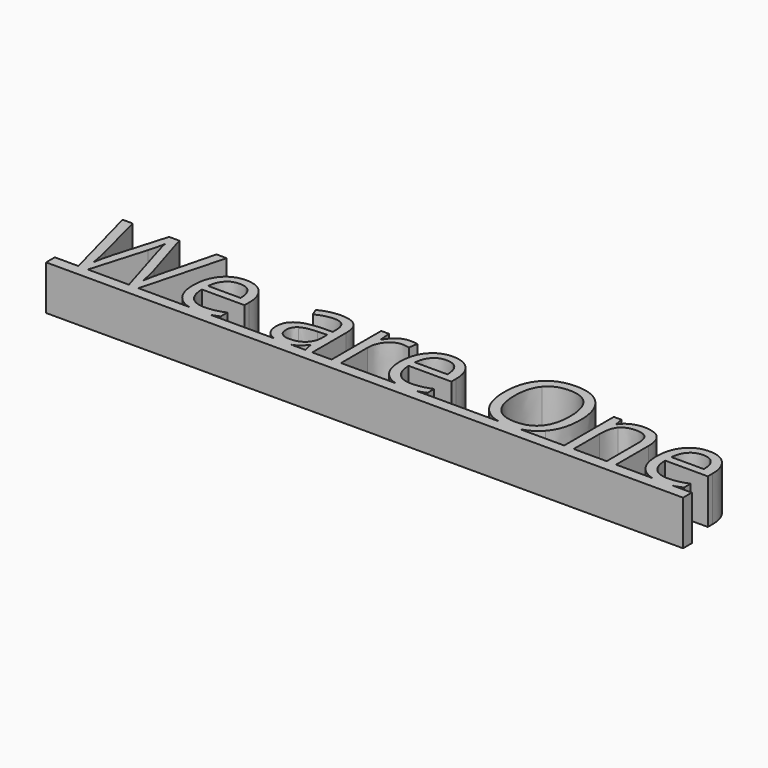
from build123d import *

# Parameters (mm, degrees)
F1_DEPTH = 7


with BuildPart() as f1:
    # F0 (on Top) → F1 (new body)
    with BuildSketch(Plane.XY):
        with BuildLine():
            Line((39.0246675003, -11.7085370013), (39.3173809253, -13.0953734228))
            Line((39.3173809253, -13.0953734228), (40.4115039218, -13.0953734228))
            Line((40.4115039218, -13.0953734228), (40.4115039218, -6.4510628623))
            add(Edge.make_bspline(
                [(39.5717289985, -3.9743662612), (40.4115039218, -4.7459361146), (40.4115039218, -6.4510628623)],
                knots=[0, 0, 0, 1, 1, 1], degree=2))
            add(Edge.make_bspline(
                [(36.9927247925, -3.2027964079), (38.7319540753, -3.2027964079), (39.5717289985, -3.9743662612)],
                knots=[0, 0, 0, 1, 1, 1], degree=2))
            add(Edge.make_bspline(
                [(35.2719677163, -3.4244628851), (36.128793907, -3.2027964079), (36.9927247925, -3.2027964079)],
                knots=[0, 0, 0, 1, 1, 1], degree=2))
            add(Edge.make_bspline(
                [(33.6961464136, -4.0354666364), (34.4151415255, -3.6461293623), (35.2719677163, -3.4244628851)],
                knots=[0, 0, 0, 1, 1, 1], degree=2))
            Line((33.6961464136, -4.0354666364), (34.1508468796, -5.1636921678))
            add(Edge.make_bspline(
                [(36.9017846993, -4.4191201546), (35.6854609526, -4.4191201546), (34.1508468796, -5.1636921678)],
                knots=[0, 0, 0, 1, 1, 1], degree=2))
            add(Edge.make_bspline(
                [(38.479026941, -4.9647607139), (37.9873820621, -4.4191201546), (36.9017846993, -4.4191201546)],
                knots=[0, 0, 0, 1, 1, 1], degree=2))
            add(Edge.make_bspline(
                [(38.9706718199, -6.6556780721), (38.9706718199, -5.5104012732), (38.479026941, -4.9647607139)],
                knots=[0, 0, 0, 1, 1, 1], degree=2))
            Line((38.9706718199, -6.6556780721), (38.9706718199, -7.2609980675))
            Line((38.9706718199, -7.2609980675), (37.3195407525, -7.3149937479))
            add(Edge.make_bspline(
                [(32.604865295, -10.4041150392), (32.604865295, -7.4570876435), (37.3195407525, -7.3149937479)],
                knots=[0, 0, 0, 1, 1, 1], degree=2))
            add(Edge.make_bspline(
                [(33.4261680118, -12.5269978402), (32.604865295, -11.7795839491), (32.604865295, -10.4041150392)],
                knots=[0, 0, 0, 1, 1, 1], degree=2))
            add(Edge.make_bspline(
                [(34.4278100444, -13.0953734228), (33.8454988608, -12.9086034224), (33.4261680118, -12.5269978402)],
                knots=[0.4894320446, 0.4894320446, 0.4894320446, 1, 1, 1], degree=2))
            Line((34.4278100444, -13.0953734228), (37.1051414676, -13.0953734228))
            add(Edge.make_bspline(
                [(37.5028418779, -12.9490167102), (37.3160728416, -13.0330444299), (37.1051414676, -13.0953734228)],
                knots=[0, 0, 0, 0.2582329607, 0.2582329607, 0.2582329607], degree=2))
            add(Edge.make_bspline(
                [(38.9536205525, -11.7085370013), (38.2260998068, -12.6236216892), (37.5028418779, -12.9490167102)],
                knots=[0, 0, 0, 1, 1, 1], degree=2))
            Line((38.9536205525, -11.7085370013), (39.0246675003, -11.7085370013))
        make_face()
        with BuildLine():
            add(Edge.make_bspline(
                [(35.9867000114, -12.0552461066), (37.3650107991, -12.0552461066), (38.1507900421, -11.3007275207)],
                knots=[0, 0, 0, 1, 1, 1], degree=2))
            add(Edge.make_bspline(
                [(34.6339661248, -11.6389109924), (35.11708537, -12.0552461066), (35.9867000114, -12.0552461066)],
                knots=[0, 0, 0, 1, 1, 1], degree=2))
            add(Edge.make_bspline(
                [(34.1508468796, -10.4211663067), (34.1508468796, -11.2225758781), (34.6339661248, -11.6389109924)],
                knots=[0, 0, 0, 1, 1, 1], degree=2))
            add(Edge.make_bspline(
                [(34.9266795498, -8.9163919518), (34.1508468796, -9.400932136), (34.1508468796, -10.4211663067)],
                knots=[0, 0, 0, 1, 1, 1], degree=2))
            add(Edge.make_bspline(
                [(37.4616346482, -8.3693304536), (35.7025122201, -8.4318517676), (34.9266795498, -8.9163919518)],
                knots=[0, 0, 0, 1, 1, 1], degree=2))
            Line((37.4616346482, -8.3693304536), (38.936569285, -8.3096510174))
            Line((38.936569285, -8.3096510174), (38.936569285, -9.1877912925))
            add(Edge.make_bspline(
                [(38.1507900421, -11.3007275207), (38.936569285, -10.5462089349), (38.936569285, -9.1877912925)],
                knots=[0, 0, 0, 1, 1, 1], degree=2))
        make_face(mode=Mode.SUBTRACT)
        with BuildLine():
            Line((40.4115039218, -13.0953734228), (39.3173809253, -13.0953734228))
            Line((39.3173809253, -13.0953734228), (37.1051414676, -13.0953734228))
            add(Edge.make_bspline(
                [(37.1051414676, -13.0953734228), (36.499246928, -13.2744117313), (35.6939865863, -13.2744117313)],
                knots=[0.2582329607, 0.2582329607, 0.2582329607, 1, 1, 1], degree=2))
            add(Edge.make_bspline(
                [(35.6939865863, -13.2744117313), (34.9860153726, -13.2744117313), (34.4278100444, -13.0953734228)],
                knots=[0, 0, 0, 0.4894320446, 0.4894320446, 0.4894320446], degree=2))
            Line((34.4278100444, -13.0953734228), (24.3351313223, -13.0953734228))
            add(Edge.make_bspline(
                [(24.3351313223, -13.0953734228), (24.2650180095, -13.1119319906), (24.1957485506, -13.1266340798)],
                knots=[0.9005120931, 0.9005120931, 0.9005120931, 1, 1, 1], degree=2))
            add(Edge.make_bspline(
                [(24.1957485506, -13.1266340798), (23.499488462, -13.2744117313), (22.5133568262, -13.2744117313)],
                knots=[0, 0, 0, 1, 1, 1], degree=2))
            add(Edge.make_bspline(
                [(22.5133568262, -13.2744117313), (21.7176978405, -13.2744117313), (21.0455868884, -13.0953734228)],
                knots=[0, 0, 0, 0.3688754729, 0.3688754729, 0.3688754729], degree=2))
            Line((21.0455868884, -13.0953734228), (15.2645353461, -13.0953734228))
            Line((15.2645353461, -13.0953734228), (13.1181084461, -13.0953734228))
            Line((13.1181084461, -13.0953734228), (11.6261225418, -13.0953734228))
            Line((11.6261225418, -13.0953734228), (5.1864271911, -13.0953734228))
            Line((5.1864271911, -13.0953734228), (3.6944412868, -13.0953734228))
            Line((3.6944412868, -13.0953734228), (0, -13.0953734228))
            Line((0, -13.0953734228), (0, -14.8112857714))
            Line((0, -14.8112857714), (99.9942272902, -14.8112857714))
            Line((99.9942272902, -14.8112857714), (99.9942272902, -13.0953734228))
            Line((99.9942272902, -13.0953734228), (97.0644708699, -13.0953734228))
            add(Edge.make_bspline(
                [(97.0644708699, -13.0953734228), (96.9943575571, -13.1119319906), (96.9250880982, -13.1266340798)],
                knots=[0.9005120931, 0.9005120931, 0.9005120931, 1, 1, 1], degree=2))
            add(Edge.make_bspline(
                [(96.9250880982, -13.1266340798), (96.2288280095, -13.2744117313), (95.2426963738, -13.2744117313)],
                knots=[0, 0, 0, 1, 1, 1], degree=2))
            add(Edge.make_bspline(
                [(95.2426963738, -13.2744117313), (94.447037388, -13.2744117313), (93.774926436, -13.0953734228)],
                knots=[0, 0, 0, 0.3688754729, 0.3688754729, 0.3688754729], degree=2))
            Line((93.774926436, -13.0953734228), (88.1038990565, -13.0953734228))
            Line((88.1038990565, -13.0953734228), (86.6289644197, -13.0953734228))
            Line((86.6289644197, -13.0953734228), (86.2403680865, -13.0953734228))
            Line((86.2403680865, -13.0953734228), (81.4425372286, -13.0953734228))
            Line((81.4425372286, -13.0953734228), (79.9676025918, -13.0953734228))
            Line((79.9676025918, -13.0953734228), (72.9898686268, -13.0953734228))
            add(Edge.make_bspline(
                [(72.9898686268, -13.0953734228), (72.224875064, -13.2744117313), (71.3368193702, -13.2744117313)],
                knots=[0.6833950988, 0.6833950988, 0.6833950988, 1, 1, 1], degree=2))
            add(Edge.make_bspline(
                [(71.3368193702, -13.2744117313), (70.4209187003, -13.2744117313), (69.6385356677, -13.0953734228)],
                knots=[0, 0, 0, 0.319412416, 0.319412416, 0.319412416], degree=2))
            Line((69.6385356677, -13.0953734228), (56.8064283554, -13.0953734228))
            add(Edge.make_bspline(
                [(56.8064283554, -13.0953734228), (56.7363150426, -13.1119319906), (56.6670455837, -13.1266340798)],
                knots=[0.9005120931, 0.9005120931, 0.9005120931, 1, 1, 1], degree=2))
            add(Edge.make_bspline(
                [(56.6670455837, -13.1266340798), (55.9707854951, -13.2744117313), (54.9846538593, -13.2744117313)],
                knots=[0, 0, 0, 1, 1, 1], degree=2))
            add(Edge.make_bspline(
                [(54.9846538593, -13.2744117313), (54.1889948736, -13.2744117313), (53.5168839215, -13.0953734228)],
                knots=[0, 0, 0, 0.3688754729, 0.3688754729, 0.3688754729], degree=2))
            Line((53.5168839215, -13.0953734228), (44.9215641696, -13.0953734228))
            Line((44.9215641696, -13.0953734228), (43.4466295328, -13.0953734228))
            Line((43.4466295328, -13.0953734228), (40.4115039218, -13.0953734228))
        make_face()
        with BuildLine():
            add(Edge.make_bspline(
                [(37.1051414676, -13.0953734228), (36.499246928, -13.2744117313), (35.6939865863, -13.2744117313)],
                knots=[0.2582329607, 0.2582329607, 0.2582329607, 1, 1, 1], degree=2))
            Line((37.1051414676, -13.0953734228), (34.4278100444, -13.0953734228))
            add(Edge.make_bspline(
                [(35.6939865863, -13.2744117313), (34.9860153726, -13.2744117313), (34.4278100444, -13.0953734228)],
                knots=[0, 0, 0, 0.4894320446, 0.4894320446, 0.4894320446], degree=2))
        make_face()
        with BuildLine():
            Line((43.4466295328, -3.361941571), (43.4466295328, -13.0953734228))
            Line((43.4466295328, -13.0953734228), (44.9215641696, -13.0953734228))
            Line((44.9215641696, -13.0953734228), (44.9215641696, -7.8720018188))
            add(Edge.make_bspline(
                [(45.7599181539, -5.483403433), (44.9215641696, -6.4425372286), (44.9215641696, -7.8720018188)],
                knots=[0, 0, 0, 1, 1, 1], degree=2))
            add(Edge.make_bspline(
                [(47.78049335, -4.5242696374), (46.5982721382, -4.5242696374), (45.7599181539, -5.483403433)],
                knots=[0, 0, 0, 1, 1, 1], degree=2))
            add(Edge.make_bspline(
                [(48.8461975674, -4.6578378993), (48.2437194498, -4.5242696374), (47.78049335, -4.5242696374)],
                knots=[0, 0, 0, 1, 1, 1], degree=2))
            Line((48.8461975674, -4.6578378993), (49.0508127771, -3.2908946232))
            add(Edge.make_bspline(
                [(47.8884847107, -3.1829032625), (48.5364328748, -3.1829032625), (49.0508127771, -3.2908946232)],
                knots=[0, 0, 0, 1, 1, 1], degree=2))
            add(Edge.make_bspline(
                [(46.2089348642, -3.6987041037), (46.9734000227, -3.1829032625), (47.8884847107, -3.1829032625)],
                knots=[0, 0, 0, 1, 1, 1], degree=2))
            add(Edge.make_bspline(
                [(44.9045129021, -5.1636921678), (45.4444697056, -4.2145049449), (46.2089348642, -3.6987041037)],
                knots=[0, 0, 0, 1, 1, 1], degree=2))
            Line((44.9045129021, -5.1636921678), (44.8334659543, -5.1636921678))
            Line((44.8334659543, -5.1636921678), (44.6629532795, -3.361941571))
            Line((44.6629532795, -3.361941571), (43.4466295328, -3.361941571))
        make_face()
        with BuildLine():
            add(Edge.make_bspline(
                [(24.3351313223, -13.0953734228), (24.2650180095, -13.1119319906), (24.1957485506, -13.1266340798)],
                knots=[0.9005120931, 0.9005120931, 0.9005120931, 1, 1, 1], degree=2))
            Line((24.3351313223, -13.0953734228), (21.0455868884, -13.0953734228))
            add(Edge.make_bspline(
                [(22.5133568262, -13.2744117313), (21.7176978405, -13.2744117313), (21.0455868884, -13.0953734228)],
                knots=[0, 0, 0, 0.3688754729, 0.3688754729, 0.3688754729], degree=2))
            add(Edge.make_bspline(
                [(24.1957485506, -13.1266340798), (23.499488462, -13.2744117313), (22.5133568262, -13.2744117313)],
                knots=[0, 0, 0, 1, 1, 1], degree=2))
        make_face()
        with BuildLine():
            Line((21.0455868884, -13.0953734228), (24.3351313223, -13.0953734228))
            add(Edge.make_bspline(
                [(25.6735250654, -12.6435148346), (24.9697600728, -12.9454939951), (24.3351313223, -13.0953734228)],
                knots=[0, 0, 0, 0.9005120931, 0.9005120931, 0.9005120931], degree=2))
            Line((25.6735250654, -12.6435148346), (25.6735250654, -11.3277253609))
            add(Edge.make_bspline(
                [(22.5673525065, -11.9841991588), (24.1389109924, -11.9841991588), (25.6735250654, -11.3277253609)],
                knots=[0, 0, 0, 1, 1, 1], degree=2))
            add(Edge.make_bspline(
                [(20.2540638854, -11.096112311), (21.0753666023, -11.9841991588), (22.5673525065, -11.9841991588)],
                knots=[0, 0, 0, 1, 1, 1], degree=2))
            add(Edge.make_bspline(
                [(19.387291122, -8.4943730817), (19.4327611686, -10.2080254632), (20.2540638854, -11.096112311)],
                knots=[0, 0, 0, 1, 1, 1], degree=2))
            Line((19.387291122, -8.4943730817), (26.0912811186, -8.4943730817))
            Line((26.0912811186, -8.4943730817), (26.0912811186, -7.5622371263))
            add(Edge.make_bspline(
                [(25.0255769012, -4.3864385586), (26.0912811186, -5.5899738547), (26.0912811186, -7.5622371263)],
                knots=[0, 0, 0, 1, 1, 1], degree=2))
            add(Edge.make_bspline(
                [(22.1325451859, -3.1829032625), (23.9598726839, -3.1829032625), (25.0255769012, -4.3864385586)],
                knots=[0, 0, 0, 1, 1, 1], degree=2))
            add(Edge.make_bspline(
                [(19.0178469933, -4.568318745), (20.1773331818, -3.1829032625), (22.1325451859, -3.1829032625)],
                knots=[0, 0, 0, 1, 1, 1], degree=2))
            add(Edge.make_bspline(
                [(17.8583608048, -8.3096510174), (17.8583608048, -5.9537342276), (19.0178469933, -4.568318745)],
                knots=[0, 0, 0, 1, 1, 1], degree=2))
            add(Edge.make_bspline(
                [(19.1073661476, -11.9586222576), (17.8583608048, -10.6428327839), (17.8583608048, -8.3096510174)],
                knots=[0, 0, 0, 1, 1, 1], degree=2))
            add(Edge.make_bspline(
                [(21.0455868884, -13.0953734228), (19.8956440539, -12.789049267), (19.1073661476, -11.9586222576)],
                knots=[0.3688754729, 0.3688754729, 0.3688754729, 1, 1, 1], degree=2))
        make_face()
        with BuildLine():
            add(Edge.make_bspline(
                [(22.1126520405, -4.4191201546), (20.9417983403, -4.4191201546), (20.2441173127, -5.1821643742)],
                knots=[0, 0, 0, 1, 1, 1], degree=2))
            add(Edge.make_bspline(
                [(23.890246675, -5.1608502899), (23.269296351, -4.4191201546), (22.1126520405, -4.4191201546)],
                knots=[0, 0, 0, 1, 1, 1], degree=2))
            add(Edge.make_bspline(
                [(24.511196999, -7.2951006025), (24.511196999, -5.9025804251), (23.890246675, -5.1608502899)],
                knots=[0, 0, 0, 1, 1, 1], degree=2))
            Line((24.511196999, -7.2951006025), (19.4213936569, -7.2951006025))
            add(Edge.make_bspline(
                [(20.2441173127, -5.1821643742), (19.5464362851, -5.9452085938), (19.4213936569, -7.2951006025)],
                knots=[0, 0, 0, 1, 1, 1], degree=2))
        make_face(mode=Mode.SUBTRACT)
        with BuildLine():
            add(Edge.make_bspline(
                [(53.5168839215, -13.0953734228), (52.366941087, -12.789049267), (51.5786631806, -11.9586222576)],
                knots=[0.3688754729, 0.3688754729, 0.3688754729, 1, 1, 1], degree=2))
            Line((53.5168839215, -13.0953734228), (56.8064283554, -13.0953734228))
            add(Edge.make_bspline(
                [(58.1448220984, -12.6435148346), (57.4410571058, -12.9454939951), (56.8064283554, -13.0953734228)],
                knots=[0, 0, 0, 0.9005120931, 0.9005120931, 0.9005120931], degree=2))
            Line((58.1448220984, -12.6435148346), (58.1448220984, -11.3277253609))
            add(Edge.make_bspline(
                [(55.0386495396, -11.9841991588), (56.6102080255, -11.9841991588), (58.1448220984, -11.3277253609)],
                knots=[0, 0, 0, 1, 1, 1], degree=2))
            add(Edge.make_bspline(
                [(52.7253609185, -11.096112311), (53.5466636353, -11.9841991588), (55.0386495396, -11.9841991588)],
                knots=[0, 0, 0, 1, 1, 1], degree=2))
            add(Edge.make_bspline(
                [(51.8585881551, -8.4943730817), (51.9040582017, -10.2080254632), (52.7253609185, -11.096112311)],
                knots=[0, 0, 0, 1, 1, 1], degree=2))
            Line((51.8585881551, -8.4943730817), (58.5625781516, -8.4943730817))
            Line((58.5625781516, -8.4943730817), (58.5625781516, -7.5622371263))
            add(Edge.make_bspline(
                [(57.4968739343, -4.3864385586), (58.5625781516, -5.5899738547), (58.5625781516, -7.5622371263)],
                knots=[0, 0, 0, 1, 1, 1], degree=2))
            add(Edge.make_bspline(
                [(54.6038422189, -3.1829032625), (56.4311697169, -3.1829032625), (57.4968739343, -4.3864385586)],
                knots=[0, 0, 0, 1, 1, 1], degree=2))
            add(Edge.make_bspline(
                [(51.4891440264, -4.568318745), (52.6486302148, -3.1829032625), (54.6038422189, -3.1829032625)],
                knots=[0, 0, 0, 1, 1, 1], degree=2))
            add(Edge.make_bspline(
                [(50.3296578379, -8.3096510174), (50.3296578379, -5.9537342276), (51.4891440264, -4.568318745)],
                knots=[0, 0, 0, 1, 1, 1], degree=2))
            add(Edge.make_bspline(
                [(51.5786631806, -11.9586222576), (50.3296578379, -10.6428327839), (50.3296578379, -8.3096510174)],
                knots=[0, 0, 0, 1, 1, 1], degree=2))
        make_face()
        with BuildLine():
            add(Edge.make_bspline(
                [(54.5839490735, -4.4191201546), (53.4130953734, -4.4191201546), (52.7154143458, -5.1821643742)],
                knots=[0, 0, 0, 1, 1, 1], degree=2))
            add(Edge.make_bspline(
                [(56.3615437081, -5.1608502899), (55.7405933841, -4.4191201546), (54.5839490735, -4.4191201546)],
                knots=[0, 0, 0, 1, 1, 1], degree=2))
            add(Edge.make_bspline(
                [(56.9824940321, -7.2951006025), (56.9824940321, -5.9025804251), (56.3615437081, -5.1608502899)],
                knots=[0, 0, 0, 1, 1, 1], degree=2))
            Line((56.9824940321, -7.2951006025), (51.89269069, -7.2951006025))
            add(Edge.make_bspline(
                [(52.7154143458, -5.1821643742), (52.0177333182, -5.9452085938), (51.89269069, -7.2951006025)],
                knots=[0, 0, 0, 1, 1, 1], degree=2))
        make_face(mode=Mode.SUBTRACT)
        with BuildLine():
            Line((56.8064283554, -13.0953734228), (53.5168839215, -13.0953734228))
            add(Edge.make_bspline(
                [(54.9846538593, -13.2744117313), (54.1889948736, -13.2744117313), (53.5168839215, -13.0953734228)],
                knots=[0, 0, 0, 0.3688754729, 0.3688754729, 0.3688754729], degree=2))
            add(Edge.make_bspline(
                [(56.6670455837, -13.1266340798), (55.9707854951, -13.2744117313), (54.9846538593, -13.2744117313)],
                knots=[0, 0, 0, 1, 1, 1], degree=2))
            add(Edge.make_bspline(
                [(56.8064283554, -13.0953734228), (56.7363150426, -13.1119319906), (56.6670455837, -13.1266340798)],
                knots=[0.9005120931, 0.9005120931, 0.9005120931, 1, 1, 1], degree=2))
        make_face()
        with BuildLine():
            add(Edge.make_bspline(
                [(69.6385356677, -13.0953734228), (67.9714740531, -12.7138877831), (66.9105945209, -11.51955212)],
                knots=[0.319412416, 0.319412416, 0.319412416, 1, 1, 1], degree=2))
            Line((69.6385356677, -13.0953734228), (72.9898686268, -13.0953734228))
            add(Edge.make_bspline(
                [(75.718995112, -11.488291463), (74.6411154944, -12.7089173001), (72.9898686268, -13.0953734228)],
                knots=[0, 0, 0, 0.6833950988, 0.6833950988, 0.6833950988], degree=2))
            add(Edge.make_bspline(
                [(77.2962373536, -6.5846311242), (77.2962373536, -9.7021711947), (75.718995112, -11.488291463)],
                knots=[0, 0, 0, 1, 1, 1], degree=2))
            add(Edge.make_bspline(
                [(75.7246788678, -1.6823917245), (77.2962373536, -3.45856542), (77.2962373536, -6.5846311242)],
                knots=[0, 0, 0, 1, 1, 1], degree=2))
            add(Edge.make_bspline(
                [(71.3538706377, 0.0937819711), (74.1531203819, 0.0937819711), (75.7246788678, -1.6823917245)],
                knots=[0, 0, 0, 1, 1, 1], degree=2))
            add(Edge.make_bspline(
                [(66.9148573377, -1.6511310674), (68.4778901898, 0.0937819711), (71.3538706377, 0.0937819711)],
                knots=[0, 0, 0, 1, 1, 1], degree=2))
            add(Edge.make_bspline(
                [(65.3518244856, -6.5675798568), (65.3518244856, -3.3960441059), (66.9148573377, -1.6511310674)],
                knots=[0, 0, 0, 1, 1, 1], degree=2))
            add(Edge.make_bspline(
                [(66.9105945209, -11.51955212), (65.3518244856, -9.7646925088), (65.3518244856, -6.5675798568)],
                knots=[0, 0, 0, 1, 1, 1], degree=2))
        make_face()
        with BuildLine():
            add(Edge.make_bspline(
                [(66.9489598727, -6.5846311242), (66.9489598727, -9.2218938274), (68.0729225872, -10.5859952256)],
                knots=[0, 0, 0, 1, 1, 1], degree=2))
            add(Edge.make_bspline(
                [(68.0729225872, -2.6202114357), (66.9489598727, -3.9843128339), (66.9489598727, -6.5846311242)],
                knots=[0, 0, 0, 1, 1, 1], degree=2))
            add(Edge.make_bspline(
                [(71.3538706377, -1.2561100375), (69.1968853018, -1.2561100375), (68.0729225872, -2.6202114357)],
                knots=[0, 0, 0, 1, 1, 1], degree=2))
            add(Edge.make_bspline(
                [(74.5992952143, -2.610264863), (73.5023303399, -1.2561100375), (71.3538706377, -1.2561100375)],
                knots=[0, 0, 0, 1, 1, 1], degree=2))
            add(Edge.make_bspline(
                [(75.6962600887, -6.5846311242), (75.6962600887, -3.9644196885), (74.5992952143, -2.610264863)],
                knots=[0, 0, 0, 1, 1, 1], degree=2))
            add(Edge.make_bspline(
                [(74.5950323974, -10.5916789815), (75.6962600887, -9.2332613391), (75.6962600887, -6.5846311242)],
                knots=[0, 0, 0, 1, 1, 1], degree=2))
            add(Edge.make_bspline(
                [(71.3368193702, -11.9500966238), (73.4938047061, -11.9500966238), (74.5950323974, -10.5916789815)],
                knots=[0, 0, 0, 1, 1, 1], degree=2))
            add(Edge.make_bspline(
                [(68.0729225872, -10.5859952256), (69.1968853018, -11.9500966238), (71.3368193702, -11.9500966238)],
                knots=[0, 0, 0, 1, 1, 1], degree=2))
        make_face(mode=Mode.SUBTRACT)
        with BuildLine():
            Line((72.9898686268, -13.0953734228), (69.6385356677, -13.0953734228))
            add(Edge.make_bspline(
                [(71.3368193702, -13.2744117313), (70.4209187003, -13.2744117313), (69.6385356677, -13.0953734228)],
                knots=[0, 0, 0, 0.319412416, 0.319412416, 0.319412416], degree=2))
            add(Edge.make_bspline(
                [(72.9898686268, -13.0953734228), (72.224875064, -13.2744117313), (71.3368193702, -13.2744117313)],
                knots=[0.6833950988, 0.6833950988, 0.6833950988, 1, 1, 1], degree=2))
        make_face()
        with BuildLine():
            Line((11.6261225418, -13.0953734228), (13.1181084461, -13.0953734228))
            Line((13.1181084461, -13.0953734228), (16.5908832557, -0.1108332386))
            Line((16.5908832557, -0.1108332386), (14.9909059907, -0.1108332386))
            Line((14.9909059907, -0.1108332386), (12.9475957713, -8.1135614414))
            add(Edge.make_bspline(
                [(12.3081732409, -11.1856314653), (12.4786859157, -9.9238376719), (12.9475957713, -8.1135614414)],
                knots=[0, 0, 0, 1, 1, 1], degree=2))
            add(Edge.make_bspline(
                [(11.5891781289, -8.0766170285), (12.0154598158, -9.4549278163), (12.3081732409, -11.1856314653)],
                knots=[0, 0, 0, 1, 1, 1], degree=2))
            Line((11.5891781289, -8.0766170285), (9.1480050017, -0.1108332386))
            Line((9.1480050017, -0.1108332386), (7.5480277367, -0.1108332386))
            Line((7.5480277367, -0.1108332386), (5.223371604, -8.0055700807))
            add(Edge.make_bspline(
                [(4.5129021257, -11.1856314653), (4.7516198704, -9.5600772991), (5.223371604, -8.0055700807)],
                knots=[0, 0, 0, 1, 1, 1], degree=2))
            add(Edge.make_bspline(
                [(3.8905308628, -8.1306127089), (4.3168125497, -9.8186881892), (4.5129021257, -11.1856314653)],
                knots=[0, 0, 0, 1, 1, 1], degree=2))
            Line((3.8905308628, -8.1306127089), (1.8386950097, -0.1108332386))
            Line((1.8386950097, -0.1108332386), (0.2387177447, -0.1108332386))
            Line((0.2387177447, -0.1108332386), (3.6944412868, -13.0953734228))
            Line((3.6944412868, -13.0953734228), (5.1864271911, -13.0953734228))
            Line((5.1864271911, -13.0953734228), (7.7270660452, -4.4532226896))
            add(Edge.make_bspline(
                [(8.3494373082, -1.8870069342), (8.1533477322, -3.0607025122), (7.7270660452, -4.4532226896)],
                knots=[0, 0, 0, 1, 1, 1], degree=2))
            add(Edge.make_bspline(
                [(8.5881550529, -2.9441855178), (8.3579629419, -2.0660452427), (8.3494373082, -1.8870069342)],
                knots=[0, 0, 0, 1, 1, 1], degree=2))
            add(Edge.make_bspline(
                [(9.0059111061, -4.4020688871), (8.8183471638, -3.8223257929), (8.5881550529, -2.9441855178)],
                knots=[0, 0, 0, 1, 1, 1], degree=2))
            Line((9.0059111061, -4.4020688871), (11.6261225418, -13.0953734228))
        make_face()
        with BuildLine():
            Line((79.9676025918, -3.361941571), (79.9676025918, -13.0953734228))
            Line((79.9676025918, -13.0953734228), (81.4425372286, -13.0953734228))
            Line((81.4425372286, -13.0953734228), (81.4425372286, -7.9885188132))
            add(Edge.make_bspline(
                [(82.1530067068, -5.2617369558), (81.4425372286, -6.0873024895), (81.4425372286, -7.9885188132)],
                knots=[0, 0, 0, 1, 1, 1], degree=2))
            add(Edge.make_bspline(
                [(84.3895646243, -4.4361714221), (82.8634761851, -4.4361714221), (82.1530067068, -5.2617369558)],
                knots=[0, 0, 0, 1, 1, 1], degree=2))
            add(Edge.make_bspline(
                [(86.0875866773, -5.0230192111), (85.5462089349, -4.4361714221), (84.3895646243, -4.4361714221)],
                knots=[0, 0, 0, 1, 1, 1], degree=2))
            add(Edge.make_bspline(
                [(86.6289644197, -6.7977719677), (86.6289644197, -5.6098670001), (86.0875866773, -5.0230192111)],
                knots=[0, 0, 0, 1, 1, 1], degree=2))
            Line((86.6289644197, -6.7977719677), (86.6289644197, -13.0953734228))
            Line((86.6289644197, -13.0953734228), (88.1038990565, -13.0953734228))
            Line((88.1038990565, -13.0953734228), (88.1038990565, -6.7466181653))
            add(Edge.make_bspline(
                [(87.2158122087, -4.0312038195), (88.1038990565, -4.8795043765), (88.1038990565, -6.7466181653)],
                knots=[0, 0, 0, 1, 1, 1], degree=2))
            add(Edge.make_bspline(
                [(84.5686029328, -3.1829032625), (86.3277253609, -3.1829032625), (87.2158122087, -4.0312038195)],
                knots=[0, 0, 0, 1, 1, 1], degree=2))
            add(Edge.make_bspline(
                [(82.7483801296, -3.5793452313), (83.5654200296, -3.1829032625), (84.5686029328, -3.1829032625)],
                knots=[0, 0, 0, 1, 1, 1], degree=2))
            add(Edge.make_bspline(
                [(81.4766397636, -4.6947823122), (81.9313402296, -3.9757872002), (82.7483801296, -3.5793452313)],
                knots=[0, 0, 0, 1, 1, 1], degree=2))
            Line((81.4766397636, -4.6947823122), (81.4055928157, -4.6947823122))
            Line((81.4055928157, -4.6947823122), (81.166875071, -3.361941571))
            Line((81.166875071, -3.361941571), (79.9676025918, -3.361941571))
        make_face()
        with BuildLine():
            add(Edge.make_bspline(
                [(93.774926436, -13.0953734228), (92.6249836015, -12.789049267), (91.8367056951, -11.9586222576)],
                knots=[0.3688754729, 0.3688754729, 0.3688754729, 1, 1, 1], degree=2))
            Line((93.774926436, -13.0953734228), (97.0644708699, -13.0953734228))
            add(Edge.make_bspline(
                [(98.4028646129, -12.6435148346), (97.6990996203, -12.9454939951), (97.0644708699, -13.0953734228)],
                knots=[0, 0, 0, 0.9005120931, 0.9005120931, 0.9005120931], degree=2))
            Line((98.4028646129, -12.6435148346), (98.4028646129, -11.3277253609))
            add(Edge.make_bspline(
                [(95.2966920541, -11.9841991588), (96.86825054, -11.9841991588), (98.4028646129, -11.3277253609)],
                knots=[0, 0, 0, 1, 1, 1], degree=2))
            add(Edge.make_bspline(
                [(92.983403433, -11.096112311), (93.8047061498, -11.9841991588), (95.2966920541, -11.9841991588)],
                knots=[0, 0, 0, 1, 1, 1], degree=2))
            add(Edge.make_bspline(
                [(92.1166306695, -8.4943730817), (92.1621007162, -10.2080254632), (92.983403433, -11.096112311)],
                knots=[0, 0, 0, 1, 1, 1], degree=2))
            Line((92.1166306695, -8.4943730817), (98.8206206661, -8.4943730817))
            Line((98.8206206661, -8.4943730817), (98.8206206661, -7.5622371263))
            add(Edge.make_bspline(
                [(97.7549164488, -4.3864385586), (98.8206206661, -5.5899738547), (98.8206206661, -7.5622371263)],
                knots=[0, 0, 0, 1, 1, 1], degree=2))
            add(Edge.make_bspline(
                [(94.8618847334, -3.1829032625), (96.6892122314, -3.1829032625), (97.7549164488, -4.3864385586)],
                knots=[0, 0, 0, 1, 1, 1], degree=2))
            add(Edge.make_bspline(
                [(91.7471865409, -4.568318745), (92.9066727293, -3.1829032625), (94.8618847334, -3.1829032625)],
                knots=[0, 0, 0, 1, 1, 1], degree=2))
            add(Edge.make_bspline(
                [(90.5877003524, -8.3096510174), (90.5877003524, -5.9537342276), (91.7471865409, -4.568318745)],
                knots=[0, 0, 0, 1, 1, 1], degree=2))
            add(Edge.make_bspline(
                [(91.8367056951, -11.9586222576), (90.5877003524, -10.6428327839), (90.5877003524, -8.3096510174)],
                knots=[0, 0, 0, 1, 1, 1], degree=2))
        make_face()
        with BuildLine():
            add(Edge.make_bspline(
                [(94.841991588, -4.4191201546), (93.6711378879, -4.4191201546), (92.9734568603, -5.1821643742)],
                knots=[0, 0, 0, 1, 1, 1], degree=2))
            add(Edge.make_bspline(
                [(96.6195862226, -5.1608502899), (95.9986358986, -4.4191201546), (94.841991588, -4.4191201546)],
                knots=[0, 0, 0, 1, 1, 1], degree=2))
            add(Edge.make_bspline(
                [(97.2405365466, -7.2951006025), (97.2405365466, -5.9025804251), (96.6195862226, -5.1608502899)],
                knots=[0, 0, 0, 1, 1, 1], degree=2))
            Line((97.2405365466, -7.2951006025), (92.1507332045, -7.2951006025))
            add(Edge.make_bspline(
                [(92.9734568603, -5.1821643742), (92.2757758327, -5.9452085938), (92.1507332045, -7.2951006025)],
                knots=[0, 0, 0, 1, 1, 1], degree=2))
        make_face(mode=Mode.SUBTRACT)
        with BuildLine():
            Line((97.0644708699, -13.0953734228), (93.774926436, -13.0953734228))
            add(Edge.make_bspline(
                [(95.2426963738, -13.2744117313), (94.447037388, -13.2744117313), (93.774926436, -13.0953734228)],
                knots=[0, 0, 0, 0.3688754729, 0.3688754729, 0.3688754729], degree=2))
            add(Edge.make_bspline(
                [(96.9250880982, -13.1266340798), (96.2288280095, -13.2744117313), (95.2426963738, -13.2744117313)],
                knots=[0, 0, 0, 1, 1, 1], degree=2))
            add(Edge.make_bspline(
                [(97.0644708699, -13.0953734228), (96.9943575571, -13.1119319906), (96.9250880982, -13.1266340798)],
                knots=[0.9005120931, 0.9005120931, 0.9005120931, 1, 1, 1], degree=2))
        make_face()
    extrude(amount=F1_DEPTH)


solid = f1.part
